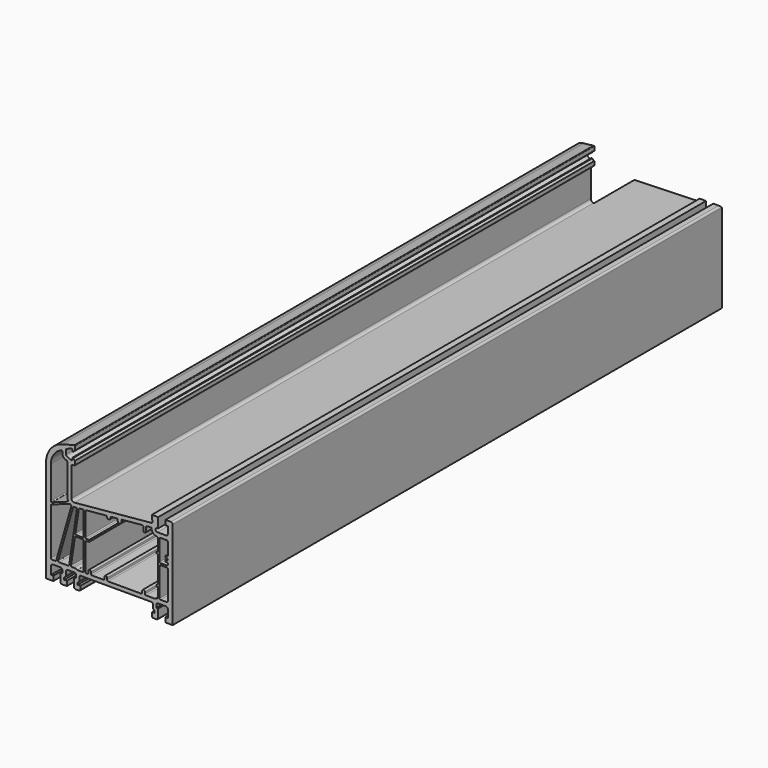
from build123d import *

# Parameters (mm, degrees)
F1_DEPTH = 10000
F3_DEPTH = 4500


# Not quite as in the source:
# - ends of sketch curves that miss each other by under 0.0002 mm in the source are joined


with BuildPart() as f1:
    # F0 (on Front) → F1 (new body)
    with BuildSketch(Plane.XZ):
        with BuildLine():
            Line((-889, 548.5347424), (-889, -889))
            Line((-889, -889), (-787.4, -889))
            Line((-787.4, -889), (-787.4, -822.96))
            Line((-787.4, -822.96), (-820.42, -822.96))
            Line((-820.42, -822.96), (-820.42, -711.2))
            ThreePointArc((-820.42, -711.2), (-812.9805122421, -693.2394877579), (-795.02, -685.8))
            Line((-795.02, -685.8), (-685.8, -685.8))
            ThreePointArc((-685.8, -685.8), (-667.8394877579, -693.2394877579), (-660.4, -711.2))
            Line((-660.4, -711.2), (-660.4, -749.3))
            Line((-660.4, -749.3), (-685.8, -749.3))
            Line((-685.8, -749.3), (-685.8, -876.3))
            Line((-685.8, -876.3), (-673.1, -889))
            Line((-673.1, -889), (-596.9, -889))
            Line((-596.9, -889), (-596.9, -822.96))
            Line((-596.9, -822.96), (-635, -822.96))
            Line((-635, -822.96), (-635, -793.2940954))
            ThreePointArc((-635, -793.2940954), (-616.4059100987, -774.7000010582), (-609.6, -749.3))
            Line((-609.6, -749.3), (-609.6, -711.2))
            ThreePointArc((-609.6, -711.2), (-602.1605122421, -693.2394877579), (-584.2, -685.8))
            Line((-584.2, -685.8), (-495.3, -685.8))
            ThreePointArc((-495.3, -685.8), (-482.6000022205, -689.2029534619), (-473.3029573079, -698.499995559))
            ThreePointArc((-473.3029573079, -698.499995559), (-470.7654846759, -704.6259937777), (-469.9, -711.2))
            Line((-469.9, -711.2), (-469.9, -749.3))
            Line((-469.9, -749.3), (-495.3, -749.3))
            Line((-495.3, -749.3), (-495.3, -876.3))
            Line((-495.3, -876.3), (-482.6, -889))
            Line((-482.6, -889), (-419.1, -889))
            Line((-419.1, -889), (-406.4, -876.3))
            Line((-406.4, -876.3), (-406.4, -822.96))
            Line((-406.4, -822.96), (-444.5, -822.96))
            Line((-444.5, -822.96), (-444.5, -793.2940954))
            ThreePointArc((-444.5, -793.2940954), (-425.9059100987, -774.7000010582), (-419.1, -749.3))
            Line((-419.1, -749.3), (-419.1, -711.2))
            ThreePointArc((-419.1, -711.2), (-415.3802561211, -702.2197438789), (-406.4, -698.5))
            Line((-406.4, -698.5), (596.9, -698.5))
            ThreePointArc((596.9, -698.5), (605.8802561211, -702.2197438789), (609.6, -711.2))
            Line((609.6, -711.2), (609.6, -749.3))
            ThreePointArc((609.6, -749.3), (616.4059100987, -774.7000010582), (635.0000021165, -793.2940917342))
            Line((635.0000021165, -793.2940917342), (635, -822.96))
            Line((635, -822.96), (596.9, -822.96))
            Line((596.9, -822.96), (596.9, -876.3))
            Line((596.9, -876.3), (609.6, -889))
            Line((609.6, -889), (673.1, -889))
            Line((673.1, -889), (685.8, -876.3))
            Line((685.8, -876.3), (685.8, -749.3))
            Line((685.8, -749.3), (660.4, -749.3))
            Line((660.4, -749.3), (660.4, -711.2))
            ThreePointArc((660.4, -711.2), (661.2654830324, -704.6259999114), (663.8029509579, -698.5000065575))
            ThreePointArc((663.8029509579, -698.5000065575), (673.0999967213, -689.2029566369), (685.8, -685.8))
            Line((685.8, -685.8), (795.02, -685.8))
            ThreePointArc((795.02, -685.8), (812.9805122421, -693.2394877579), (820.42, -711.2))
            Line((820.42, -711.2), (820.42, -822.96))
            Line((820.42, -822.96), (787.4, -822.96))
            Line((787.4, -822.96), (787.4, -889))
            Line((787.4, -889), (889, -889))
            Line((889, -889), (889, 355.6))
            ThreePointArc((889, 355.6), (881.5605122421, 373.5605122421), (863.6, 381))
            Line((863.6, 381), (787.4, 381))
            Line((787.4, 381), (787.4, 314.96))
            Line((787.4, 314.96), (820.42, 314.96))
            Line((820.42, 314.96), (820.42, 215.9))
            ThreePointArc((820.42, 215.9), (812.9805122421, 197.9394877579), (795.02, 190.5))
            Line((795.02, 190.5), (673.1, 190.5))
            ThreePointArc((673.1, 190.5), (655.7827591038, 197.3184724056), (647.7629299549, 214.1131363983))
            ThreePointArc((647.7629299549, 214.1131363983), (654.5184724056, 233.2172408962), (673.1, 241.3))
            Line((673.1, 241.3), (685.8, 241.3))
            Line((685.8, 241.3), (685.8, 381))
            Line((685.8, 381), (596.9, 381))
            Line((596.9, 381), (604.5809092, 293.2068812))
            ThreePointArc((604.5809092, 293.2068812), (601.6825015075, 283.9658746444), (593.1121497834, 279.4552090875))
            Line((593.1121497834, 279.4552090875), (572.9650466, 277.570438))
            Line((572.9650466, 277.570438), (-491.7512136, 177.9656334))
            ThreePointArc((-491.7512136, 177.9656334), (-520.9554302247, 187.7324850229), (-533.4, 215.9))
            Line((-533.4, 215.9), (-533.4, 622.3))
            ThreePointArc((-533.4, 622.3), (-529.6802561211, 631.2802561211), (-520.7, 635))
            Line((-520.7, 635), (-495.3, 635))
            ThreePointArc((-495.3, 635), (-486.3197438789, 638.7197438789), (-482.6, 647.7))
            Line((-482.6, 647.7), (-482.6, 698.5))
            Line((-482.6, 698.5), (-508, 723.9))
            Line((-508, 723.9), (-520.7, 723.9))
            Line((-520.7, 723.9), (-520.7, 701.04))
            ThreePointArc((-520.7, 701.04), (-526.5763029291, 690.3289235702), (-538.7672690212, 689.5298990771))
            Line((-538.7672690212, 689.5298990771), (-602.2672486, 719.140421))
            ThreePointArc((-602.2672486, 719.140421), (-607.6110764298, 723.8268355291), (-609.6, 730.6505326))
            Line((-609.6, 730.6505326), (-609.6, 793.3494674))
            ThreePointArc((-609.6, 793.3494674), (-607.6110764298, 800.1731644709), (-602.2672690212, 804.8595683229))
            Line((-602.2672690212, 804.8595683229), (-538.7672486, 834.4701116))
            ThreePointArc((-538.7672486, 834.4701116), (-526.5763029291, 833.6710764298), (-520.7, 822.96))
            Line((-520.7, 822.96), (-520.7, 800.1))
            Line((-520.7, 800.1), (-508, 800.1))
            Line((-508, 800.1), (-482.6, 825.5))
            Line((-482.6, 825.5), (-482.6, 881.38))
            ThreePointArc((-482.6, 881.38), (-485.5812400415, 887.4253540878), (-492.1922063117, 888.7403534062))
            Line((-492.1922063117, 888.7403534062), (-663.0880312, 842.9489364))
            ThreePointArc((-663.0880312, 842.9489364), (-826.0141013776, 734.0852217174), (-889, 548.5347424))
        make_face()
        with BuildLine():
            ThreePointArc((-820.42, 37.410517), (-818.1232380904, 44.694927562), (-812.0636791755, 49.3446047833))
            Line((-812.0636791755, 49.3446047833), (-561.1497794, 140.669772))
            ThreePointArc((-561.1497794, 140.669772), (-555.1255930563, 141.3240040218), (-549.4839701069, 139.1123902964))
            ThreePointArc((-549.4839701069, 139.1123902964), (-545.1404408941, 136.2245906727), (-540.6433693867, 133.5822057349))
            ThreePointArc((-540.6433693867, 133.5822057349), (-535.0440503822, 127.3338720048), (-534.5628196657, 118.9575675147))
            Line((-534.5628196657, 118.9575675147), (-746.6621084, -620.7206026))
            ThreePointArc((-746.6621084, -620.7206026), (-751.227090517, -627.3626751304), (-758.8701358, -629.92))
            Line((-758.8701358, -629.92), (-807.72, -629.92))
            ThreePointArc((-807.72, -629.92), (-816.7002561211, -626.2002561211), (-820.42, -617.22))
            Line((-820.42, -617.22), (-820.42, 37.410517))
        make_face(mode=Mode.SUBTRACT)
        with BuildLine():
            ThreePointArc((-373.38, -236.22), (-364.3997438789, -239.9397438789), (-360.68, -248.92))
            Line((-360.68, -248.92), (-360.68, -629.92))
            ThreePointArc((-360.68, -629.92), (-364.3997438789, -638.9002561211), (-373.38, -642.62))
            Line((-373.38, -642.62), (-448.1215828, -642.62))
            ThreePointArc((-448.1215828, -642.62), (-451.4227999147, -642.1834402009), (-454.497059757, -640.9037741041))
            ThreePointArc((-454.497059757, -640.9037741041), (-474.172274712, -632.7139654196), (-495.3, -629.92))
            Line((-495.3, -629.92), (-525.998821, -629.92))
            ThreePointArc((-525.998821, -629.92), (-535.619898632, -625.5100461518), (-538.5593214093, -615.3428134171))
            Line((-538.5593214093, -615.3428134171), (-483.5165336, -247.0428384))
            ThreePointArc((-483.5165336, -247.0428384), (-479.2460765518, -239.298922368), (-470.9560304, -236.22))
            Line((-470.9560304, -236.22), (-373.38, -236.22))
        make_face(mode=Mode.SUBTRACT)
        with BuildLine():
            ThreePointArc((-497.4246847824, 121.9440203362), (-491.9799440726, 121.9786625487), (-486.5463475014, 122.3285622215))
            Line((-486.5463475014, 122.3285622215), (-469.6735336, 123.9070166))
            ThreePointArc((-469.6735336, 123.9070166), (-459.266492708, 119.9918270332), (-455.9301049456, 109.3850459039))
            Line((-455.9301049456, 109.3850459039), (-564.8025026, -619.097187))
            ThreePointArc((-564.8025026, -619.097187), (-569.0729610703, -626.8410788574), (-577.3630058, -629.92))
            Line((-577.3630058, -629.92), (-706.0229212, -629.92))
            ThreePointArc((-706.0229212, -629.92), (-716.1655942237, -624.8630480787), (-718.2309428641, -613.7193990447))
            Line((-718.2309428641, -613.7193990447), (-509.9198082, 112.7478568))
            ThreePointArc((-509.9198082, 112.7478568), (-505.2396905609, 119.4756741479), (-497.4246847824, 121.9440203362))
        make_face(mode=Mode.SUBTRACT)
        with BuildLine():
            ThreePointArc((-428.9586008093, 118.0126921829), (-425.1276925966, 125.3596164016), (-417.5810299631, 128.7802941569))
            Line((-417.5810299631, 128.7802941569), (-374.5629288, 132.804662))
            ThreePointArc((-374.5629288, 132.804662), (-364.8281933327, 129.5490563628), (-360.68, 120.1598816))
            Line((-360.68, 120.1598816), (-360.68, -203.2))
            ThreePointArc((-360.68, -203.2), (-364.3997438789, -212.1802561211), (-373.38, -215.9))
            Line((-373.38, -215.9), (-464.1231256, -215.9))
            ThreePointArc((-464.1231256, -215.9), (-473.744203232, -211.4900461518), (-476.6836260093, -201.3228134171))
            Line((-476.6836260093, -201.3228134171), (-428.9586008093, 118.0126921829))
        make_face(mode=Mode.SUBTRACT)
        with BuildLine():
            ThreePointArc((668.02, -482.6), (677.0002561211, -486.3197438789), (680.72, -495.3))
            Line((680.72, -495.3), (680.72, -618.917228))
            ThreePointArc((680.72, -618.917228), (677.8129607122, -627.0035077682), (670.4226896868, -631.3878768311))
            ThreePointArc((670.4226896868, -631.3878768311), (657.3097586954, -635.0767804779), (644.997043561, -640.9037899611))
            ThreePointArc((644.997043561, -640.9037899611), (641.9228147085, -642.183443056), (638.6216082, -642.62))
            Line((638.6216082, -642.62), (511.81, -642.62))
            ThreePointArc((511.81, -642.62), (502.8297438789, -638.9002561211), (499.11, -629.92))
            Line((499.11, -629.92), (499.11, -603.25))
            ThreePointArc((499.11, -603.25), (480.06, -584.2), (461.01, -603.25))
            Line((461.01, -603.25), (461.01, -629.92))
            ThreePointArc((461.01, -629.92), (457.2902561211, -638.9002561211), (448.31, -642.62))
            Line((448.31, -642.62), (-19.05, -642.62))
            ThreePointArc((-19.05, -642.62), (-28.0302561211, -638.9002561211), (-31.75, -629.92))
            Line((-31.75, -629.92), (-31.75, -603.25))
            ThreePointArc((-31.75, -603.25), (-50.8, -584.2), (-69.85, -603.25))
            Line((-69.85, -603.25), (-69.85, -629.92))
            ThreePointArc((-69.85, -629.92), (-73.5697438789, -638.9002561211), (-82.55, -642.62))
            Line((-82.55, -642.62), (-245.11, -642.62))
            ThreePointArc((-245.11, -642.62), (-254.0902561211, -638.9002561211), (-257.81, -629.92))
            Line((-257.81, -629.92), (-257.81, -603.25))
            ThreePointArc((-257.81, -603.25), (-276.86, -584.2), (-295.91, -603.25))
            Line((-295.91, -603.25), (-295.91, -629.92))
            ThreePointArc((-295.91, -629.92), (-299.6297438789, -638.9002561211), (-308.61, -642.62))
            Line((-308.61, -642.62), (-322.58, -642.62))
            ThreePointArc((-322.58, -642.62), (-331.5602561211, -638.9002561211), (-335.28, -629.92))
            Line((-335.28, -629.92), (-335.28, -254))
            ThreePointArc((-335.28, -254), (-331.5602561211, -245.0197438789), (-322.58, -241.3))
            Line((-322.58, -241.3), (-284.48, -241.3))
            Line((-284.48, -241.3), (-284.48, -215.9))
            Line((-284.48, -215.9), (-322.58, -215.9))
            ThreePointArc((-322.58, -215.9), (-331.5602561211, -212.1802561211), (-335.28, -203.2))
            Line((-335.28, -203.2), (-335.28, 124.912247))
            ThreePointArc((-335.28, 124.912247), (-331.9691747628, 133.4640536673), (-323.7629295631, 137.5570355569))
            Line((-323.7629295631, 137.5570355569), (-49.3993932, 163.2239052))
            ThreePointArc((-49.3993932, 163.2239052), (-39.8915292411, 160.1700041853), (-35.5309766074, 151.1860585939))
            ThreePointArc((-35.5309766074, 151.1860585939), (-7.7941470622, 127.1104223073), (14.9959046097, 155.9128995528))
            ThreePointArc((14.9959046097, 155.9128995528), (17.6144767278, 165.5497316378), (26.3909294369, 170.3141201569))
            Line((26.3909294369, 170.3141201569), (102.9570712, 177.4769374))
            ThreePointArc((102.9570712, 177.4769374), (112.6918066673, 174.2213063628), (116.84, 164.8321316))
            Line((116.84, 164.8321316), (116.84, 152.4))
            ThreePointArc((116.84, 152.4), (142.24, 127), (167.64, 152.4))
            Line((167.64, 152.4), (167.64, 171.9606924))
            ThreePointArc((167.64, 171.9606924), (170.9508252372, 180.5124990673), (179.1570704369, 184.6054809569))
            Line((179.1570704369, 184.6054809569), (462.3670712, 211.0999334))
            ThreePointArc((462.3670712, 211.0999334), (472.1018066673, 207.8443277628), (476.25, 198.455153))
            Line((476.25, 198.455153), (476.25, 146.05))
            ThreePointArc((476.25, 146.05), (495.3, 127), (514.35, 146.05))
            Line((514.35, 146.05), (514.35, 204.3956034))
            ThreePointArc((514.35, 204.3956034), (517.6608252372, 212.9474100673), (525.8670704369, 217.0403919569))
            Line((525.8670704369, 217.0403919569), (578.169913, 221.9333636))
            ThreePointArc((578.169913, 221.9333636), (587.5688806647, 218.9729368373), (592.0213758685, 210.1820285292))
            ThreePointArc((592.0213758685, 210.1820285292), (616.0974599888, 157.959091893), (668.7064863025, 134.7388304829))
            ThreePointArc((668.7064863025, 134.7388304829), (677.239771412, 130.7915637247), (680.72, 122.0573886))
            Line((680.72, 122.0573886), (680.72, -38.1))
            ThreePointArc((680.72, -38.1), (677.0002561211, -47.0802561211), (668.02, -50.8))
            Line((668.02, -50.8), (665.48, -50.8))
            Line((665.48, -50.8), (665.48, -76.2))
            Line((665.48, -76.2), (668.02, -76.2))
            ThreePointArc((668.02, -76.2), (677.0002561211, -79.9197438789), (680.72, -88.9))
            Line((680.72, -88.9), (680.72, -444.5))
            ThreePointArc((680.72, -444.5), (677.0002561211, -453.4802561211), (668.02, -457.2))
            Line((668.02, -457.2), (665.48, -457.2))
            Line((665.48, -457.2), (665.48, -482.6))
            Line((665.48, -482.6), (668.02, -482.6))
        make_face(mode=Mode.SUBTRACT)
        with BuildLine():
            ThreePointArc((807.72, -203.2), (816.7002561211, -206.9197438789), (820.42, -215.9))
            Line((820.42, -215.9), (820.42, -617.22))
            ThreePointArc((820.42, -617.22), (816.7002561211, -626.2002561211), (807.72, -629.92))
            Line((807.72, -629.92), (718.82, -629.92))
            ThreePointArc((718.82, -629.92), (709.8397438789, -626.2002561211), (706.12, -617.22))
            Line((706.12, -617.22), (706.12, -215.9))
            ThreePointArc((706.12, -215.9), (709.8397438789, -206.9197438789), (718.82, -203.2))
            Line((718.82, -203.2), (807.72, -203.2))
        make_face(mode=Mode.SUBTRACT)
        with BuildLine():
            ThreePointArc((718.82, -177.8), (709.8397438789, -174.0802561211), (706.12, -165.1))
            Line((706.12, -165.1), (706.12, 121.92))
            ThreePointArc((706.12, 121.92), (709.8397438789, 130.9002561211), (718.82, 134.62))
            Line((718.82, 134.62), (807.72, 134.62))
            ThreePointArc((807.72, 134.62), (816.7002561211, 130.9002561211), (820.42, 121.92))
            Line((820.42, 121.92), (820.42, -50.8))
            ThreePointArc((820.42, -50.8), (816.7002561211, -59.7802561211), (807.72, -63.5))
            Line((807.72, -63.5), (787.4, -63.5))
            Line((787.4, -63.5), (787.4, -88.9))
            Line((787.4, -88.9), (807.72, -88.9))
            ThreePointArc((807.72, -88.9), (816.7002561211, -92.6197438789), (820.42, -101.6))
            ThreePointArc((820.42, -101.6), (816.7002561211, -110.5802561211), (807.72, -114.3))
            Line((807.72, -114.3), (787.4, -114.3))
            Line((787.4, -114.3), (787.4, -139.7))
            Line((787.4, -139.7), (807.72, -139.7))
            ThreePointArc((807.72, -139.7), (816.7002561211, -143.4197438789), (820.42, -152.4))
            Line((820.42, -152.4), (820.42, -165.1))
            ThreePointArc((820.42, -165.1), (816.7002561211, -174.0802561211), (807.72, -177.8))
            Line((807.72, -177.8), (718.82, -177.8))
        make_face(mode=Mode.SUBTRACT)
        with BuildLine():
            ThreePointArc((-596.6127518422, 660.4520944516), (-591.2689297546, 655.7656905784), (-589.28, 648.9419838))
            Line((-589.28, 648.9419838), (-589.28, 635))
            Line((-589.28, 635), (-589.28, 215.9))
            ThreePointArc((-589.28, 215.9), (-586.9776386334, 195.2251124644), (-580.1833629579, 175.5632290216))
            ThreePointArc((-580.1833629579, 175.5632290216), (-579.9032005162, 165.2949796419), (-587.3104304532, 158.1782130533))
            Line((-587.3104304532, 158.1782130533), (-803.376346, 79.5366456))
            ThreePointArc((-803.376346, 79.5366456), (-815.0044203378, 81.0675027548), (-820.42, 91.470734))
            Line((-820.42, 91.470734), (-820.42, 548.5347424))
            ThreePointArc((-820.42, 548.5347424), (-781.6753507544, 678.1625721451), (-678.1511468594, 765.2674589054))
            ThreePointArc((-678.1511468594, 765.2674589054), (-666.130764467, 764.2321366649), (-660.4, 753.6151806))
            Line((-660.4, 753.6151806), (-660.4, 730.6505326))
            ThreePointArc((-660.4, 730.6505326), (-650.4553602952, 696.532012942), (-623.736271381, 673.0999936072))
            Line((-623.736271381, 673.0999936072), (-596.6127518422, 660.4520944516))
        make_face(mode=Mode.SUBTRACT)
    extrude(amount=F1_DEPTH)

    # F2 (on face) → F3 (cut, symmetric)
    with BuildSketch(Plane(origin=(0, 0, -698.5), x_dir=(1, 0, 0), z_dir=(0, 0, -1))):
        with BuildLine():
            Line((-889, 0), (889, 0))
            Line((889, 0), (889, 355.6))
            ThreePointArc((889, 355.6), (881.5605122421, 373.5605122421), (863.6, 381))
            Line((863.6, 381), (787.4, 381))
            Line((787.4, 381), (596.9, 381))
            Line((596.9, 381), (596.9, 280.4131869739))
            ThreePointArc((596.9, 280.4131869739), (595.043135271, 279.7876610723), (593.1121497834, 279.4552090875))
            Line((593.1121497834, 279.4552090875), (572.9650466, 277.570438))
            Line((572.9650466, 277.570438), (-482.6, 178.821734576))
            Line((-482.6, 178.821734576), (-482.6, 647.7))
            Line((-482.6, 647.7), (-482.6, 698.5))
            Line((-482.6, 698.5), (-482.6, 825.5))
            Line((-482.6, 825.5), (-482.6, 881.38))
            ThreePointArc((-482.6, 881.38), (-485.5812400415, 887.4253540878), (-492.1922063117, 888.7403534062))
            Line((-492.1922063117, 888.7403534062), (-663.0880312, 842.9489364))
            ThreePointArc((-663.0880312, 842.9489364), (-826.0141013776, 734.0852217174), (-889, 548.5347424))
            Line((-889, 548.5347424), (-889, 0))
        make_face()
    extrude(amount=F3_DEPTH, both=True, mode=Mode.SUBTRACT)


solid = f1.part
